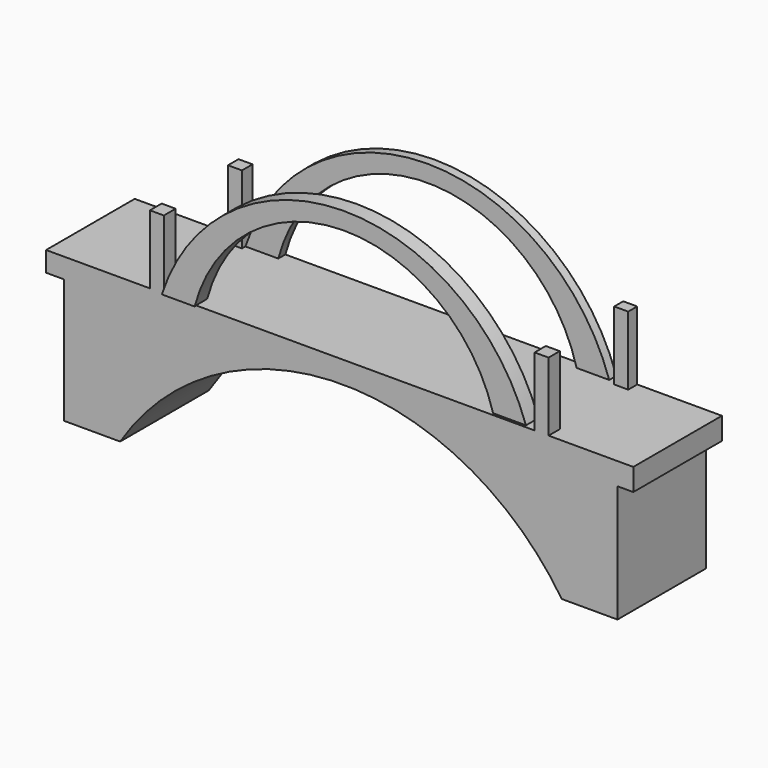
from build123d import *

# Parameters (mm, degrees)
F3_W      = 127
F3_H      = 25.4
F4_DEPTH  = 5.08
F5_W      = 3.2020173967
F5_H      = 2.5810918153
F5_H_2    = 3.2004
F5_W_2    = 3.2004
F5_H_3    = 3.030332116
F5_H_4    = 3.370467884
F6_DEPTH  = 15.748
F9_DEPTH  = 25.4
F10_DEPTH = 7.62
F13_DEPTH = 3.556
F14_DEPTH = 2.032


with BuildPart() as f4:
    # F3 (on offset) → F4 (new body)
    with BuildSketch(Plane.XY.offset(50.8)):
        with Locations((3.1030103564, 0.0919504733)):
            Rectangle(F3_W, F3_H)
    extrude(amount=F4_DEPTH)

    # F5 (on face) → F6 (join)
    with BuildSketch(Plane.XY.offset(55.88)):
        with Locations((45.5839950591, 11.5014045656)):
            Rectangle(F5_W, F5_H)
        with Locations((45.5839950591, -11.0078495267)):
            Rectangle(F5_W, F5_H_2)
        with Locations((-42.6142088447, 11.2767844153)):
            Rectangle(F5_W_2, F5_H_3)
        with Locations((-42.6142088447, -10.9228155847)):
            Rectangle(F5_W_2, F5_H_4)
    extrude(amount=F6_DEPTH)

    # F8 (on offset) → F9 (join)
    with BuildSketch(Plane(origin=(0, 12.7919504733, 0), x_dir=(-1, 0, 0), z_dir=(0, 1, 0))):
        with BuildLine():
            Line((63.9144031451, 22.7373477172), (63.9144031451, 51.2869477172))
            Line((63.9144031451, 51.2869477172), (-62.980983232, 51.2869477172))
            Line((-62.980983232, 51.2869477172), (-62.980983232, 23.8919413011))
            Line((-62.980983232, 23.8919413011), (-50.2015098581, 23.8919413011))
            ThreePointArc((-50.2015098581, 23.8919413011), (0.729046025, 50.8523148548), (51.0314504165, 22.7373477172))
            Line((51.0314504165, 22.7373477172), (63.9144031451, 22.7373477172))
        make_face()
    extrude(amount=-F9_DEPTH)

    # F10 (add): a face of the model
    f10_faces = [f4.faces().sort_by_distance(p)[0] for p in [
        (-60.3969896436, 0.0919504733, 53.5834738586),
    ]]
    extrude(f10_faces, amount=F10_DEPTH)

    # F12 (on offset) → F13 (join)
    with BuildSketch(Plane.XZ.offset(12.954)):
        with BuildLine():
            Line((34.7522422671, 56.4973130822), (42.2758869827, 56.4973130822))
            ThreePointArc((42.2758869827, 56.4973130822), (0.279509926, 86.2029094565), (-41.2007495761, 55.7807758451))
            Line((-41.2007495761, 55.7807758451), (-33.6771048605, 55.7807758451))
            ThreePointArc((-33.6771048605, 55.7807758451), (0.264117723, 82.2536287212), (34.7522422671, 56.4973130822))
        make_face()
    extrude(amount=-F13_DEPTH)


with BuildPart() as f14:
    # F11 (on offset) → F14 (new body)
    with BuildSketch(Plane(origin=(0, 12.7919504733, 0), x_dir=(-1, 0, 0), z_dir=(0, 1, 0))):
        with BuildLine():
            Line((33.4876855967, 55.8397546411), (41.0189045158, 55.8397546411))
            ThreePointArc((41.0189045158, 55.8397546411), (-0.6087174648, 86.1564382353), (-42.3918627203, 56.0544617474))
            Line((-42.3918627203, 56.0544617474), (-34.9106043577, 56.0544617474))
            ThreePointArc((-34.9106043577, 56.0544617474), (-0.6287310234, 82.3015137584), (33.4876855967, 55.8397546411))
        make_face()
    extrude(amount=-F14_DEPTH)


solid = Compound([f4.part, f14.part])
